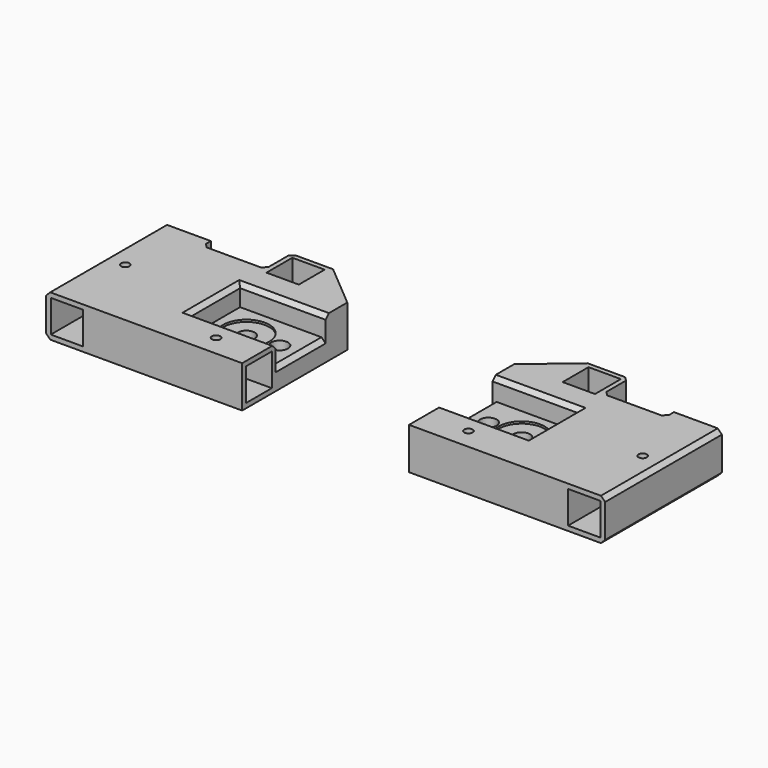
from build123d import *

# Parameters (mm, degrees)
F0_W      = 41
F0_H      = 30
F0_R      = 11
F0_R_2    = 4
F1_DEPTH  = 10
F0_W_2    = 15.5
F0_H_2    = 15.5
F0_H_3    = 20
F0_R_3    = 2
F2_DEPTH  = 20
F0_R_4    = 10
F3_DEPTH  = 2
F4_W      = 15.5
F4_H      = 15.5
F5_DEPTH  = 49
F7_START  = -1
F6_R      = 11
F7_DEPTH  = 7
F8_DEPTH  = 25
F9_W      = 15.5
F9_H      = 15.5
F10_DEPTH = 80.751
F11_SIZE  = 2
F12_R     = 5
F12_R_2   = 2
F13_DEPTH = 17
F14_DEPTH = 41


# Not quite as in the source:
# - a feature names something its author has since deleted; it is built from what else it names


with BuildPart() as f1:
    # F0 (on Top) → F1 (new body)
    with BuildSketch(Plane.XY):
        with Locations((-60.5, 0)):
            Rectangle(F0_W, F0_H)
        with Locations((-66, 0)):
            Circle(F0_R, mode=Mode.SUBTRACT)
        with Locations((-50, 0)):
            Circle(F0_R_2, mode=Mode.SUBTRACT)
    extrude(amount=F1_DEPTH)

    # F0 (on Top) → F2 (join)
    with BuildSketch(Plane.XY):
        Polygon((-81, 30), (-81, 15), (-40, 15), (-40, 28), (-61, 28), (-61, 45.75), (-81, 45.75), (-81, 35), align=None)
        with Locations((-71, 35.75)):
            Rectangle(F0_W_2, F0_H_2, mode=Mode.SUBTRACT)
        with Locations((-60.5, -25)):
            Rectangle(F0_W, F0_H_3)
        with Locations((-60.5, -25)):
            Circle(F0_R_3, mode=Mode.SUBTRACT)
        Polygon((-81, -15), (-81, 15), (-81, 30), (-111, 30), (-111, 35), (-134, 35), (-134, -35), (-81, -35), align=None)
        with Locations((-124, 0)):
            Rectangle(F0_W_2, F0_H_2, mode=Mode.SUBTRACT)
        with Locations((-124, 0)):
            Rectangle(F0_W_2, F0_H_2)
        with Locations((-124, 0)):
            Circle(F0_R_3, mode=Mode.SUBTRACT)
        Polygon((-61, 28), (-40, 28), (-61, 45.75), align=None)
    extrude(amount=F2_DEPTH)

    # F0 (on Top) → F3 (join)
    with BuildSketch(Plane.XY):
        with Locations((-66, 0)):
            Circle(F0_R)
        with Locations((-66, 0)):
            Circle(F0_R_4, mode=Mode.SUBTRACT)
    extrude(amount=F3_DEPTH)

    # F4 (on face) → F5 (cut)
    with BuildSketch(Plane.YZ.offset(-40)):
        with Locations((-25, 10)):
            Rectangle(F4_W, F4_H)
    extrude(amount=-F5_DEPTH, mode=Mode.SUBTRACT)

    # F9 (on face) → F10 (cut, through all)
    with BuildSketch(Plane.XZ.offset(35)):
        with Locations((-124, 10)):
            Rectangle(F9_W, F9_H)
    extrude(amount=-F10_DEPTH, mode=Mode.SUBTRACT)

    # F11
    f11_edges = [f1.edges().sort_by_distance(p)[0] for p in [
        (-81, 0, 20),
        (-60.5, 15, 20),
        (-60.5, -15, 20),
        (-134, 0, 20),
        (-134, 0, 0),
        (-40, 0, 10),
        (-111, 30, 10),
        (-81, 30, 10),
        (-81, 45.75, 10),
    ]]
    chamfer(f11_edges, length=F11_SIZE)

    # F12 (on face) → F13 (cut)
    with BuildSketch(Plane.YZ.offset(-40)):
        with Locations((35.75, 10)):
            Circle(F12_R)
        with Locations((35.75, 10)):
            Circle(F12_R_2, mode=Mode.SUBTRACT)
    extrude(amount=-F13_DEPTH, mode=Mode.SUBTRACT)

    # F12 (on face) → F14 (cut)
    with BuildSketch(Plane.YZ.offset(-40)):
        with Locations((35.75, 10)):
            Circle(F12_R_2)
    extrude(amount=-F14_DEPTH, mode=Mode.SUBTRACT)


with BuildPart() as f7:
    # F6 (on face) → F7 (new body)
    with BuildSketch(Plane.XY.offset(10).offset(F7_START)):
        with Locations((-66, 0)):
            Circle(F6_R)
    extrude(amount=-F7_DEPTH)

    # F0 (on Top) → F8 (cut)
    with BuildSketch(Plane.XY):
        with Locations((-66, 0)):
            Circle(F0_R_2)
    extrude(amount=F8_DEPTH, mode=Mode.SUBTRACT)


with BuildPart() as f15_1:
    # F15: instance of F7
    add(f7.part.mirror(Plane.YZ))


with BuildPart() as f15_2:
    # F15: instance of F1
    add(f1.part.mirror(Plane.YZ))


solid = Compound([f1.part, f7.part, f15_1.part, f15_2.part])
